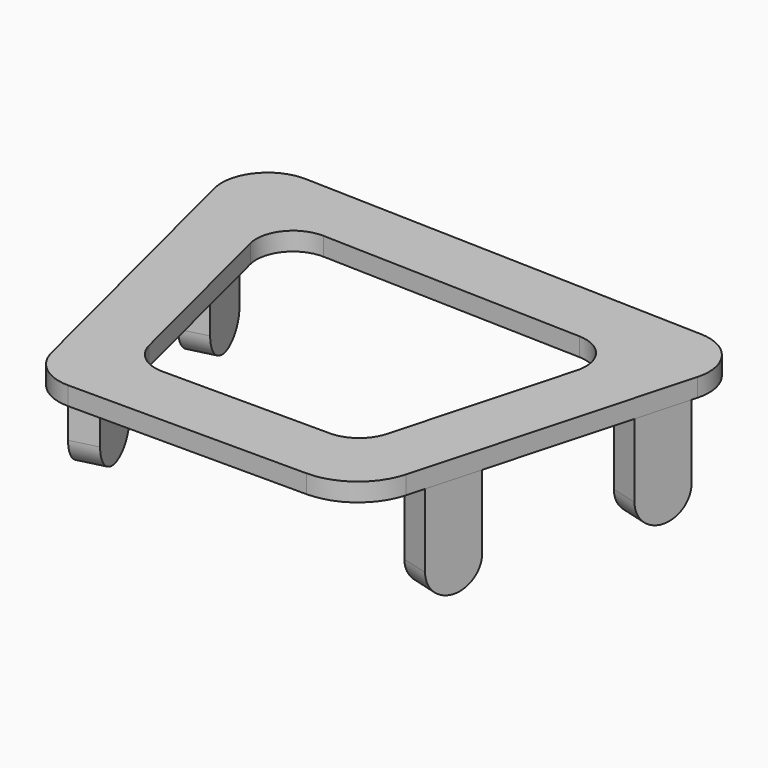
from build123d import *

# Parameters (mm, degrees)
F2_DEPTH = 2
F3_T     = 7
F4_R     = 4
F6_DEPTH = 11
F7_R     = 2.99999


# Not quite as in the source:
# - a fillet or chamfer is up to 0.001 mm smaller than in the source, because OpenCascade refuses the exact size
# - a shell that OpenCascade refuses in one call is made with other operations: the cavity is built on its own and cut out


with BuildPart() as f2:
    # F1 (on Top) → F2 (new body)
    with BuildSketch(Plane.XY):
        with BuildLine():
            ThreePointArc((-21.6449442268, 42.3033521048), (-25.6894079684, 40.4398561051), (-26.6437804137, 36.0902035288))
            Line((-26.6437804137, 36.0902035288), (-18.5483854863, 3.7846369171))
            ThreePointArc((-18.5483854863, 3.7846369171), (-16.7743151531, 1.0581212972), (-13.6983450146, 0))
            Line((-13.6983450146, 0), (12.2689166074, 0))
            ThreePointArc((12.2689166074, 0), (16.5100865033, 1.4311152002), (19.017084198, 5.1392920247))
            Line((19.017084198, 5.1392920247), (27.1577014469, 34.6625972473))
            ThreePointArc((27.1577014469, 34.6625972473), (26.3599974025, 38.9615518502), (22.4863774545, 40.9894598656))
            Line((22.4863774545, 40.9894598656), (-21.6449442268, 42.3033521048))
        make_face()
    extrude(amount=F2_DEPTH)

    # F3: shell of thickness 7, made by hand


with BuildPart() as f3_core1:
    # F3_t2: copy of F2
    add(f2.part)

    # the walls: a layer under each face that stays
    f3_faces = [f3_core1.faces().sort_by_distance(p)[0] for p in [
        (0.4207166138, 41.6464059852, 1),
        (-22.59608295, 19.937420223, 1),
        (-0.7147142036, 0, 1),
        (23.0873928224, 19.900944636, 1),
    ]]
    thicken(f3_faces, amount=-F3_T, mode=Mode.SUBTRACT)


with BuildPart() as f2_1:
    add(f2.part)

    # what is left inside the walls is the cavity
    f3_cavity = [f3_core1.part.solids().sort_by_distance(p)[0] for p in [
        (0.260689, 16.409264, 0.07),
    ]]
    add(f3_cavity, mode=Mode.SUBTRACT)

    # F4
    f4_edges = [f2_1.edges().sort_by_distance(p)[0] for p in [
        (19.732614, 34.068344, 1),
        (-19.211236, 35.227793, 1),
        (-12.137683, 7, 1),
        (12.268917, 7, 1),
    ]]
    fillet(f4_edges, radius=F4_R)

    # F5 (on face) → F6 (join)
    with BuildSketch(Plane.XY):
        Polygon((-23.3953947844, 35.4691530951), (-26.3054190674, 34.7399352453), (-24.8469833679, 28.9198866794), (-21.9369590849, 29.6491045291), align=None)
        Polygon((25.3943994744, 28.2676887604), (26.9892920247, 34.0518324094), (24.0972202001, 34.8492786846), (22.5023276498, 29.0651350355), align=None)
        Polygon((-19.3778494948, 7.0947045569), (-16.4678252118, 7.8239224066), (-17.9262609113, 13.6439709726), (-20.8362851943, 12.9147531229), align=None)
        Polygon((18.249280849, 13.6407519713), (16.6543882988, 7.8566083223), (19.5464601233, 7.0591620471), (21.1413526736, 12.8433056962), align=None)
    extrude(amount=-F6_DEPTH)

    # F7 (radius 3 in the source; OpenCascade refuses exactly that, so slightly less here)
    f7_edges = [f2_1.edges().sort_by_distance(p)[0] for p in [
        (25.543256, 34.450556, -11),
        (23.948364, 28.666412, -11),
        (19.695317, 13.242029, -11),
        (18.100424, 7.457885, -11),
        (-17.922837, 7.459313, -11),
        (-19.381273, 13.279362, -11),
        (-23.391971, 29.284496, -11),
        (-24.850407, 35.104544, -11),
    ]]
    fillet(f7_edges, radius=F7_R)


solid = f2_1.part
